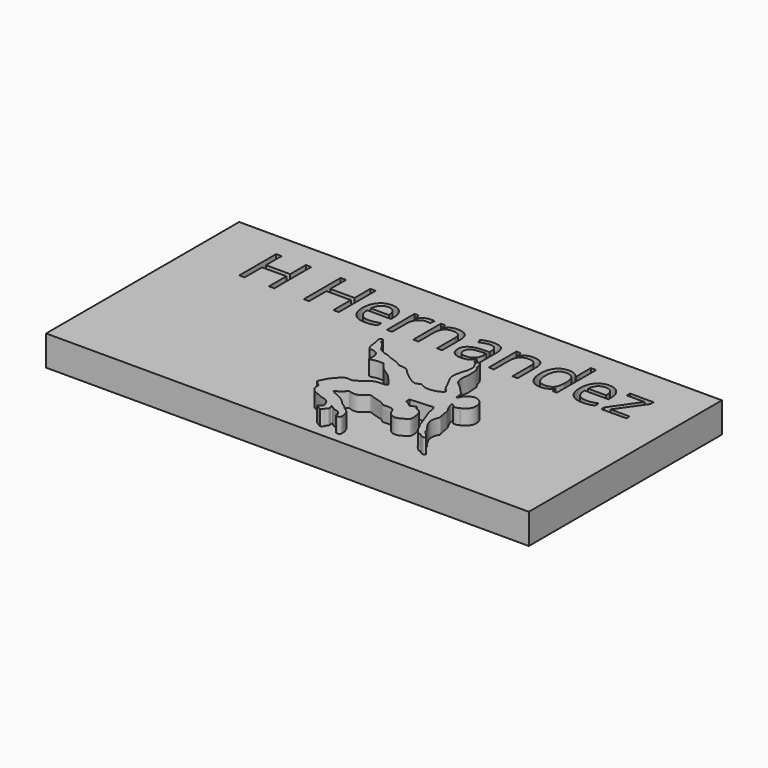
from build123d import *

# Parameters (mm, degrees)
F0_W         = 101.6
F0_H         = 50.8
F1_DEPTH     = 6.35
F2_TEXT_SIZE = 13.5908317235
F3_DEPTH     = 3.175
F4_DEPTH     = 3.175
F7_DEPTH     = 3.175


# Not quite as in the source:
# - Text() gives the source's letters only with a copy of the font that has no kerning and outlines rounded to 1/6400 em; it was checked with that copy


with BuildPart() as f1:
    # F0 (on Top) → F1 (new body)
    with BuildSketch(Plane.XY):
        with Locations((-74.7058956252, 25.4)):
            Rectangle(F0_W, F0_H)
    extrude(amount=F1_DEPTH)

    # F2 (on face) → F3 (join)
    with BuildSketch(Plane.XY.offset(6.35)):
        with Locations((-114.9461349544, 35.9757170081)):
            Text('H Hernandez', F2_TEXT_SIZE, font='Open Sans', text_align=(TextAlign.LEFT, TextAlign.BOTTOM))
    extrude(amount=-F3_DEPTH)

    # F2 (on face) → F4 (cut)
    with BuildSketch(Plane.XY.offset(6.35)):
        with Locations((-114.9461349544, 35.9757170081)):
            Text('H Hernandez', F2_TEXT_SIZE, font='Open Sans', text_align=(TextAlign.LEFT, TextAlign.BOTTOM))
    extrude(amount=-F4_DEPTH, mode=Mode.SUBTRACT)

    # F6 (on face) → F7 (join)
    with BuildSketch(Plane.XY.offset(6.35)):
        with BuildLine():
            add(Edge.make_bspline(
                [(-75.4246562719, 11.7066623643), (-74.6829429459, 12.6163249834), (-73.437083149, 14.1442900962), (-71.8144759863, 13.1395311784), (-69.1706724845, 16.1133372795), (-66.921336803, 15.6225763015), (-66.5006818781, 15.9931099031), (-66.3505420089, 16.1253605038)],
                knots=[0, 0, 0, 0, 0.2441204038, 0.4100503334, 0.6798475387, 0.8857314016, 1, 1, 1, 1], degree=3))
            add(Edge.make_bspline(
                [(-75.4246562719, 11.7066623643), (-75.8224757107, 10.9613208082), (-76.3442585623, 9.9837254354), (-76.2569913621, 9.729913341), (-75.8574362297, 9.3138657516), (-75.2198630064, 8.8290266833), (-75.1499702101, 8.9016668568), (-75.4025263256, 7.5163225096), (-74.1239897242, 6.5906542532), (-73.464512832, 6.4096716949), (-72.092881085, 5.7045707009), (-70.7698217928, 5.599754829), (-70.0291136301, 4.1237935714), (-70.1596958623, 3.3875333763), (-70.8564561546, 3.0339914628), (-70.8632958894, 2.8824929297), (-70.8341014892, 2.9210120108), (-70.8208754659, 2.9384624213)],
                knots=[0, 0, 0, 0, 0.1124844556, 0.147535425, 0.210802993, 0.2804245291, 0.2907570484, 0.3753629007, 0.473302425, 0.541411231, 0.6387480417, 0.7304399564, 0.8272536824, 0.8941876824, 0.9616474591, 0.9826250377, 1, 1, 1, 1], degree=3))
            add(Edge.make_bspline(
                [(-70.8208754659, 2.9384624213), (-70.4502115647, 2.7366837021), (-70.0795476635, 2.5349049829), (-69.7088837624, 2.3331262637)],
                knots=[0, 0, 0, 0, 1.2660795443, 1.2660795443, 1.2660795443, 1.2660795443], degree=3))
            add(Edge.make_bspline(
                [(-69.7088837624, 2.3331262637), (-69.4564021204, 2.5128120734), (-69.0912023567, 2.7727169706), (-69.2776183422, 2.9566717542), (-68.7145708512, 3.3380288926), (-68.7881304013, 3.3938450531), (-68.6794126418, 4.2578734632), (-68.9983564585, 3.9770523973), (-68.9633207691, 4.376411677), (-68.5078330369, 4.3231375636), (-68.0116842222, 3.6317104134), (-67.2348120496, 3.8104502408), (-66.0857841763, 2.8383130836), (-66.59463189, 2.1459353916), (-65.0987079639, 1.9295253793), (-65.4245889372, 3.6439725936), (-65.7784806707, 4.5344950455), (-66.9471265492, 5.1696629549), (-67.2033944577, 5.6763402653), (-68.1964447442, 6.1330676179), (-68.728969378, 6.9484519953), (-70.109382327, 7.8424947012), (-71.1727359662, 8.2427006302), (-71.7283064405, 8.4972538663), (-72.2174434733, 8.9392413117), (-70.5418794275, 9.2259445077), (-70.2218618012, 10.5207350383), (-69.7426573073, 10.2148372713), (-67.8158234182, 9.7900246237), (-66.612860564, 11.803383752), (-65.1953587688, 10.8783891041), (-63.0779276647, 10.6000026668), (-62.8227069539, 9.7735277648), (-60.5841865319, 10.2503159946), (-60.0298822876, 9.1437865435), (-59.7636406595, 8.3619926965), (-58.2772675436, 7.3504710853), (-56.6207536556, 8.4077378876), (-55.7187154079, 8.8731401761), (-55.9803823292, 10.8032863309), (-56.4859602539, 12.198160901), (-57.5286076771, 12.2164432616), (-57.6790381233, 12.9926228071), (-58.3715992299, 12.7874017646), (-58.9613065326, 12.1991586022), (-59.521773753, 13.0722595187), (-60.5598554346, 13.1866259117), (-60.4190005748, 13.872651869), (-60.3479886477, 14.218511411)],
                knots=[0, 0, 0, 0, 0.0194930483, 0.0281955312, 0.0456193484, 0.0527524779, 0.0717322231, 0.0808432415, 0.0915343106, 0.1050668441, 0.1253887721, 0.1455376133, 0.1715866509, 0.1882506356, 0.2095837424, 0.2364148475, 0.2603513615, 0.2858226064, 0.3032464732, 0.3263317638, 0.3494938236, 0.3790852711, 0.4040151748, 0.4224910975, 0.4358311819, 0.4626614477, 0.4869480039, 0.5010447236, 0.5318140148, 0.5635437162, 0.591304828, 0.6243415616, 0.6430727329, 0.6753160557, 0.6988528729, 0.7200031188, 0.748669827, 0.7799349488, 0.8018508645, 0.832921956, 0.8604607164, 0.8815971612, 0.8991387349, 0.9166928762, 0.9356463457, 0.9567712612, 0.9782062457, 1, 1, 1, 1], degree=3))
            Line((-60.3479886477, 14.218511411), (-55.6054556792, 14.5287190771))
            add(Edge.make_bspline(
                [(-55.6054556792, 14.5287190771), (-55.4988636946, 14.4548354638), (-55.1947339034, 14.2440271758), (-55.251995409, 12.815598301), (-53.8477966886, 9.7018862542), (-53.6464721012, 8.8533748356), (-53.346211872, 7.8521234651), (-52.8252140288, 7.5712919343), (-52.9621356359, 7.5147244164), (-52.9790080622, 7.5158815351), (-52.9827300663, 7.5165040336)],
                knots=[0, 0, 0, 0, 0.094141986, 0.2685634259, 0.544729963, 0.6912053898, 0.841043186, 0.9390562571, 0.9789718473, 0.9932251453, 0.9932251453, 0.9932251453, 0.9932251453], degree=3))
            add(Edge.make_bspline(
                [(-52.9827300663, 7.5165040336), (-52.8656476472, 7.2272444452), (-52.6662488777, 6.7342485264), (-52.4822105388, 6.4748129074), (-51.5335728501, 5.4945277505), (-51.3011285324, 5.8299178151), (-50.9234087931, 5.1845633499), (-49.6156986004, 4.9851038421), (-50.1961563559, 6.0169669528), (-51.1980674208, 6.6358298243), (-51.3320688281, 7.3004610567), (-51.3871668406, 7.605315569)],
                knots=[0, 0, 0, 0, 0.1161060625, 0.1977826237, 0.3387312409, 0.3946371538, 0.4969913105, 0.6204658916, 0.7307807398, 0.8741868343, 0.9940380426, 0.9940380426, 0.9940380426, 0.9940380426], degree=3))
            Line((-51.3871668406, 7.605315569), (-51.3968467634, 7.6195289851))
            add(Edge.make_bspline(
                [(-52.9247886514, 14.6924271073), (-52.7418250766, 13.5872218712), (-52.5399135154, 12.3676022437), (-52.4656221404, 12.3997494318), (-52.2354496437, 12.5195267184), (-53.7226608117, 10.4467772869), (-51.5890638472, 7.8197114733), (-51.405432909, 7.6079867844), (-51.3968467634, 7.6195289851)],
                knots=[0, 0, 0, 0, 0.2663987369, 0.2939109171, 0.3380429959, 0.5759690811, 0.8893849729, 0.9587993363, 0.9587993363, 0.9587993363, 0.9587993363], degree=3))
            add(Edge.make_bspline(
                [(-51.9400256156, 16.9933196157), (-52.04770074, 16.9267013113), (-52.3051778506, 16.7674009287), (-53.2191290264, 16.632672904), (-53.4315718859, 17.0349531269), (-53.5089648216, 17.2172778908), (-53.9444477408, 17.3082107354), (-53.8778381269, 16.9485335414), (-53.7620862989, 16.4802690631), (-53.3880459592, 15.6139475324), (-53.0796411548, 15.2225236864), (-52.9461516683, 14.9091524327), (-52.9314036596, 14.7595393689), (-52.9247886514, 14.6924271073)],
                knots=[0, 0, 0, 0, 0.092666476, 0.2215877888, 0.307330712, 0.3701120605, 0.4492344848, 0.5180534575, 0.6195703017, 0.7559573606, 0.8563756066, 0.9355739582, 1, 1, 1, 1], degree=3))
            ThreePointArc((-51.9400256156, 16.9933196157), (-50.3156926043, 19.4614984533), (-52.4632036686, 21.4909221977))
            ThreePointArc((-52.4632036686, 21.4909221977), (-53.6966305766, 20.9195161958), (-54.5147433877, 19.8339112103))
            add(Edge.make_bspline(
                [(-73.0491131544, 24.3315156549), (-72.4177161129, 24.0136292987), (-71.6509930681, 23.6276110266), (-71.617725719, 23.7392352448), (-69.4125698386, 22.9103858957), (-69.4579864727, 22.5142747432), (-67.7015415311, 22.7013808148), (-66.8266712327, 21.4285653783), (-63.2107841378, 18.6022185857), (-62.3317147773, 20.0970648071), (-60.9546454962, 18.4104022408), (-56.6334767899, 19.880156809), (-58.3119613415, 20.8406366834), (-58.6577146499, 22.1338546375), (-60.1168844611, 24.3352590592), (-60.1087937073, 25.8214859265), (-59.5373815517, 27.9370331804), (-59.3641960966, 28.1599567823), (-59.1315355916, 29.7750990832), (-59.84090501, 30.629275853), (-59.8627477271, 30.8013458756), (-60.0974825269, 31.7001367385), (-59.2921201156, 31.6253247557), (-59.4344459433, 31.2783624317), (-58.8131559639, 30.8437624797), (-59.0182263139, 30.0633626475), (-58.2332437647, 29.395114224), (-58.2781290935, 28.231836487), (-58.080346526, 26.608287449), (-58.4523813685, 25.7814314961), (-58.165944671, 23.825721566), (-57.0038972844, 23.266095545), (-55.9908731188, 21.9388983809), (-54.7975951717, 21.0742217166), (-54.9232923951, 19.3350543153), (-54.6204373533, 19.7048540775), (-54.5147433877, 19.8339112103)],
                knots=[0, 0, 0, 0, 0.0339746483, 0.0412563634, 0.0818489168, 0.0972690004, 0.1290697008, 0.1654322879, 0.2206113666, 0.2470459554, 0.2830278933, 0.3336628964, 0.360973562, 0.3938872772, 0.4373282908, 0.4723125031, 0.5112118703, 0.5269016417, 0.5608036974, 0.5884895621, 0.6009892441, 0.624119997, 0.6430143438, 0.6565728239, 0.6784495372, 0.7013722117, 0.7272171673, 0.7567155464, 0.7912088861, 0.8178276583, 0.8541645841, 0.8846010897, 0.9196010245, 0.9535276199, 0.9837815144, 1, 1, 1, 1], degree=3))
            add(Edge.make_bspline(
                [(-77.7142047882, 27.812179178), (-77.6416966238, 27.9902408346), (-77.4840471025, 28.3773880634), (-76.6928550037, 27.8544676732), (-77.0090271363, 27.2620528222), (-76.3441041866, 27.0847739372), (-75.5851886101, 25.8817090031), (-75.0325956622, 24.8357651244), (-73.2476810718, 24.2969779129), (-73.0872876552, 24.3248758056), (-73.0491131544, 24.3315156549)],
                knots=[0, 0, 0, 0, 0.0999909488, 0.2174034514, 0.3169701378, 0.4198766634, 0.5888955706, 0.7529742238, 0.941206529, 1, 1, 1, 1], degree=3))
            add(Edge.make_bspline(
                [(-71.7160999775, 21.5698294342), (-71.9373953613, 21.5626850162), (-72.3902448838, 21.5480649811), (-72.9845129821, 21.6803861603), (-74.8529476957, 21.0267037001), (-74.5291074902, 22.0454950374), (-74.6057537195, 23.4696035082), (-75.7847009006, 24.2446323222), (-77.1531063247, 24.0023636553), (-77.3946281525, 26.3310062626), (-77.6113674136, 27.3355487957), (-77.7142047882, 27.812179178)],
                knots=[0, 0, 0, 0, 0.0823775977, 0.168574035, 0.2968840212, 0.3789299251, 0.5014471907, 0.6174172753, 0.7238189068, 0.8689589582, 1, 1, 1, 1], degree=3))
            add(Edge.make_bspline(
                [(-71.7160999775, 21.5698294342), (-71.2629289769, 20.9562838099), (-70.3840039152, 19.7663121988), (-68.545299328, 18.9374915507), (-67.1533757706, 17.1540271938), (-66.3505420089, 16.1253605038)],
                knots=[0, 0, 0, 0, 0.3105700501, 0.6023505477, 1, 1, 1, 1], degree=3))
        make_face()
    extrude(amount=F7_DEPTH)


solid = f1.part
